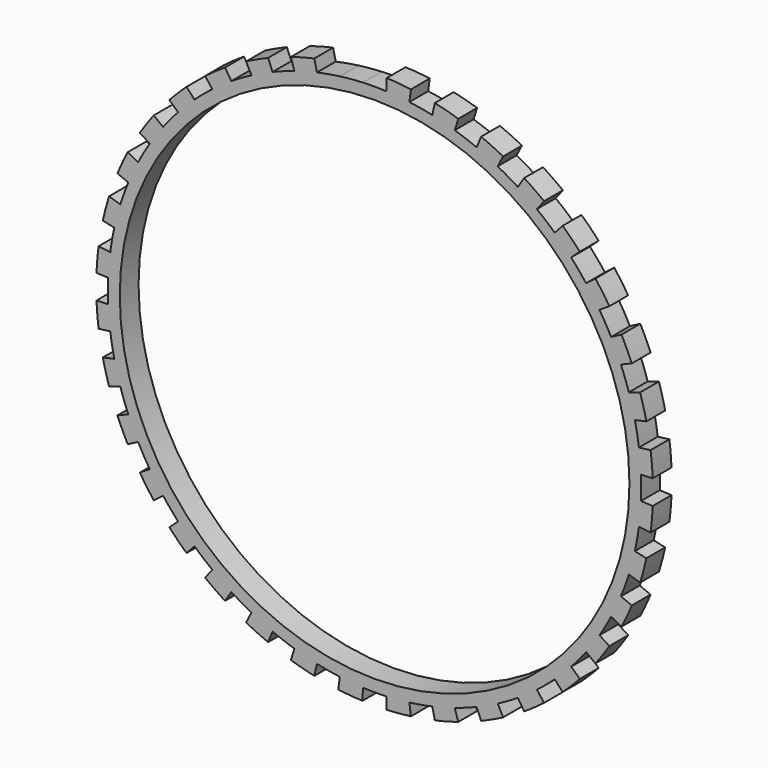
from build123d import *

# Parameters (mm, degrees)
F0_R            = 71
F0_R_2          = 65
F1_DEPTH        = 6
F3_DEPTH        = 25
F3_COPIES_COUNT = 35
F3_COPIES_ANGLE = 340
F5_DEPTH        = 25


# Not quite as in the source:
# - a pattern or mirror of a feature is missing from the dataset's text; its kind, count and spacing are read off the source's solid


with BuildPart() as f1:
    # F0 (on Front) → F1 (new body)
    with BuildSketch(Plane.XZ):
        Circle(F0_R)
        Circle(F0_R_2, mode=Mode.SUBTRACT)
    extrude(amount=F1_DEPTH)

    # F2 (on Front) → F3 (cut)
    with BuildSketch(Plane.XZ):
        with BuildLine():
            ThreePointArc((-2.9661183408, 67.9352790676), (0, 68), (2.9661183408, 67.9352790676))
            Line((2.9661183408, 67.9352790676), (3.3463516673, 76.6440540311))
            Line((3.3463516673, 76.6440540311), (-3.4023122145, 77.9257612834))
            Line((-3.4023122145, 77.9257612834), (-2.9661183408, 67.9352790676))
        make_face()
    f3 = extrude(amount=F3_DEPTH, mode=Mode.SUBTRACT)

    # F3_copies: F3 ×35 about axis
    f3_copies_axis = Axis((0, 0, 0), (0, 1, 0))
    for i in range(1, F3_COPIES_COUNT):
        add(f3.rotate(f3_copies_axis, i * F3_COPIES_ANGLE / (F3_COPIES_COUNT - 1)), mode=Mode.SUBTRACT)

    # F3_copies1: F3 across plane
    add(f3.mirror(Plane(origin=(0, 0, 0), x_dir=(0.0871557427, 0, -0.9961946981), z_dir=(-0.9961946981, 0, -0.0871557427))), mode=Mode.SUBTRACT)

    # F4 (on face) → F5 (cut)
    with BuildSketch(Plane.XZ.offset(6)):
        with BuildLine():
            Line((-9.2673596476, 70.3925851575), (-8.875781071, 67.4182505734))
            ThreePointArc((-8.875781071, 67.4182505734), (-5.9265905068, 67.7412394702), (-2.9661183408, 67.9352790676))
            Line((-2.9661183408, 67.9352790676), (-3.0969765029, 70.9324237323))
            ThreePointArc((-3.0969765029, 70.9324237323), (-6.1880577351, 70.7298235645), (-9.2673596476, 70.3925851575))
        make_face()
    extrude(amount=-F5_DEPTH, mode=Mode.SUBTRACT)


solid = f1.part
